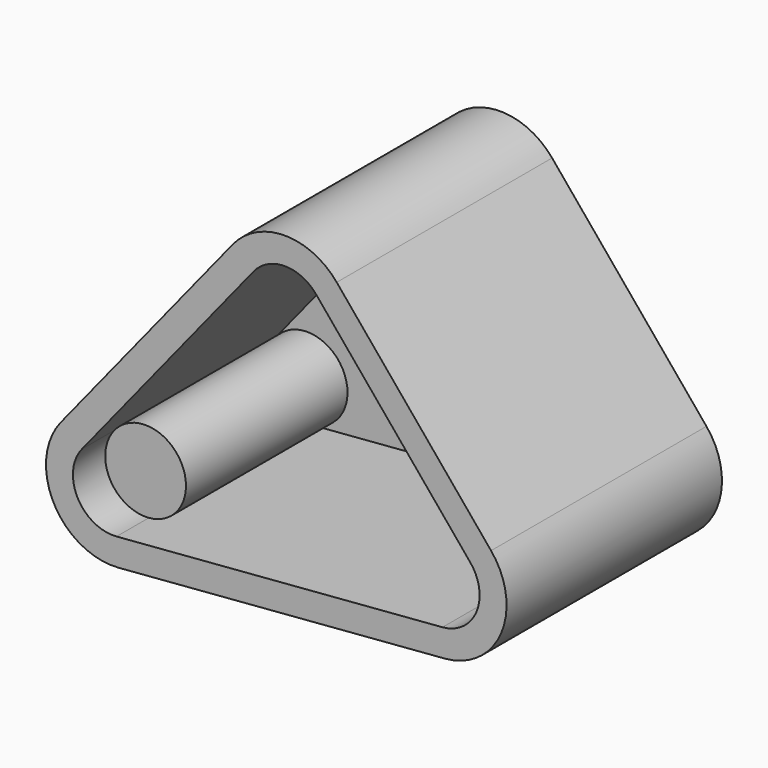
from build123d import *

# Parameters (mm, degrees)
F1_DEPTH = 25.4
F2_T     = -2.54
F3_R     = 3.81
F4_DEPTH = 19.05


# Not quite as in the source:
# - the program builds the solid bodies; features that only make, move or delete a surface that nothing else refers to are left out


with BuildPart() as f1:
    # F0 (on Front) → F1 (new body)
    with BuildSketch(Plane.XZ):
        with BuildLine():
            ThreePointArc((-12.1858643886, -0.9756983319), (-6.8419002324, 2.8860613911), (-7.8055765775, 9.4085202038))
            Line((-7.8055765775, 9.4085202038), (-22.3667159803, 26.9599173237))
            ThreePointArc((-22.3667159803, 26.9599173237), (-27.2929398052, 29.2553210157), (-32.1905035986, 26.8993863451))
            Line((-32.1905035986, 26.8993863451), (-48.3822646253, 6.8856646257))
            ThreePointArc((-48.3822646253, 6.8856646257), (-49.0625660789, -0.0700213051), (-42.9387648181, -3.4380229313))
            Line((-42.9387648181, -3.4380229313), (-12.1858643886, -0.9756983319))
        make_face()
    extrude(amount=F1_DEPTH)

    # F2
    f2_openings = [f1.faces().sort_by_distance(p)[0] for p in [
        (-28.02144, -25.4, 9.948419),
    ]]
    offset(amount=F2_T, openings=f2_openings)

    # F3 (on face) → F4 (join)
    with BuildSketch(Plane.XZ.offset(2.54)):
        with Locations((-43.4455749435, 2.8917198357)):
            Circle(F3_R)
    extrude(amount=F4_DEPTH)


solid = f1.part
